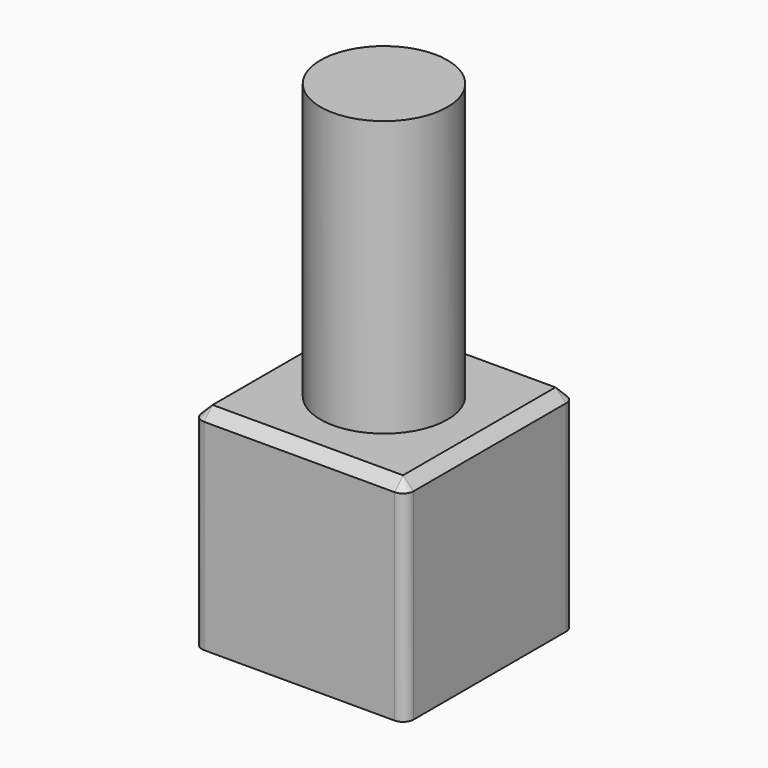
from build123d import *

# Parameters (mm, degrees)
F0_W     = 127
F0_H     = 127
F0_R     = 38.1
F1_DEPTH = 127
F2_DEPTH = 165.1
F3_R     = 6.35
F4_SIZE  = 6.34999


# Not quite as in the source:
# - a fillet or chamfer is up to 0.001 mm smaller than in the source, because OpenCascade refuses the exact size


with BuildPart() as f1:
    # F0 (on Top) → F1 (new body)
    with BuildSketch(Plane.XY):
        Rectangle(F0_W, F0_H)
        Circle(F0_R, mode=Mode.SUBTRACT)
        Circle(F0_R)
    extrude(amount=-F1_DEPTH)

    # F0 (on Top) → F2 (join)
    with BuildSketch(Plane.XY):
        Circle(F0_R)
    extrude(amount=F2_DEPTH)

    # F3
    f3_edges = [f1.edges().sort_by_distance(p)[0] for p in [
        (-63.5, -63.5, -63.5),
        (63.5, -63.5, -63.5),
        (63.5, 63.5, -63.5),
        (-63.5, 63.5, -63.5),
    ]]
    fillet(f3_edges, radius=F3_R)

    # F4 (size 6.35 in the source; OpenCascade refuses exactly that, so slightly less here)
    f4_edges = [f1.edges().sort_by_distance(p)[0] for p in [
        (0, -63.5, 0),
    ]]
    chamfer(f4_edges, length=F4_SIZE)


solid = f1.part
